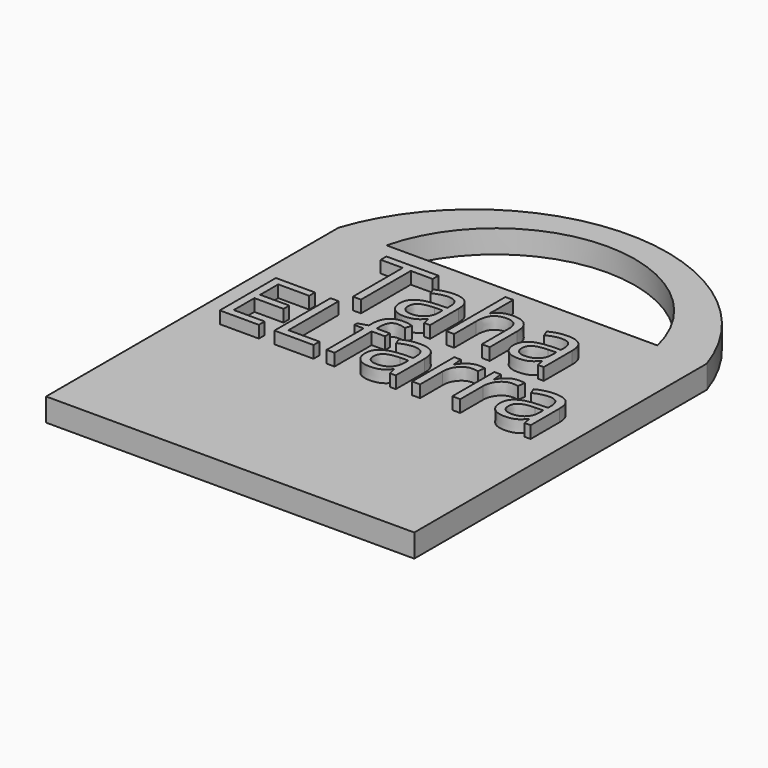
from build123d import *

# Parameters (mm, degrees)
F1_DEPTH       = 4.826
F2_TEXT_SIZE   = 20.3455332667
F2_TEXT_SIZE_2 = 20.570302796
F3_DEPTH       = 2.54


# Not quite as in the source:
# - Text() gives the source's letters only with a copy of the font that has no kerning and outlines rounded to 1/6400 em; it was checked with that copy


with BuildPart() as f1:
    # F0 (on Top) → F1 (new body)
    with BuildSketch(Plane.XY):
        with BuildLine():
            Line((-10.3067271411, 0), (0, 0))
            ThreePointArc((0, 0), (-38.5398827493, 27.7361551832), (-77.0797654986, 0))
            Line((-77.0797654986, 0), (-67.0396909118, 0))
            ThreePointArc((-67.0396909118, 0), (-38.6732090265, 22.278132075), (-10.3067271411, 0))
        make_face()
        Polygon((0, -76.5412598848), (0, 0), (-10.3067271411, 0), (-67.0396909118, 0), (-77.0797654986, 0), (-77.0797654986, -76.5412598848), align=None)
    extrude(amount=F1_DEPTH)

    # F2 (on face) → F3 (join)
    with BuildSketch(Plane.XY.offset(4.826)):
        with Locations((-61.7229012338, -21.4112722315)):
            Text('Taha', F2_TEXT_SIZE, font='Open Sans', text_align=(TextAlign.LEFT, TextAlign.BOTTOM))
        with Locations((-72.9164647491, -38.8150941581)):
            Text('ELfarra', F2_TEXT_SIZE_2, font='Open Sans', text_align=(TextAlign.LEFT, TextAlign.BOTTOM))
    extrude(amount=F3_DEPTH)


solid = f1.part
